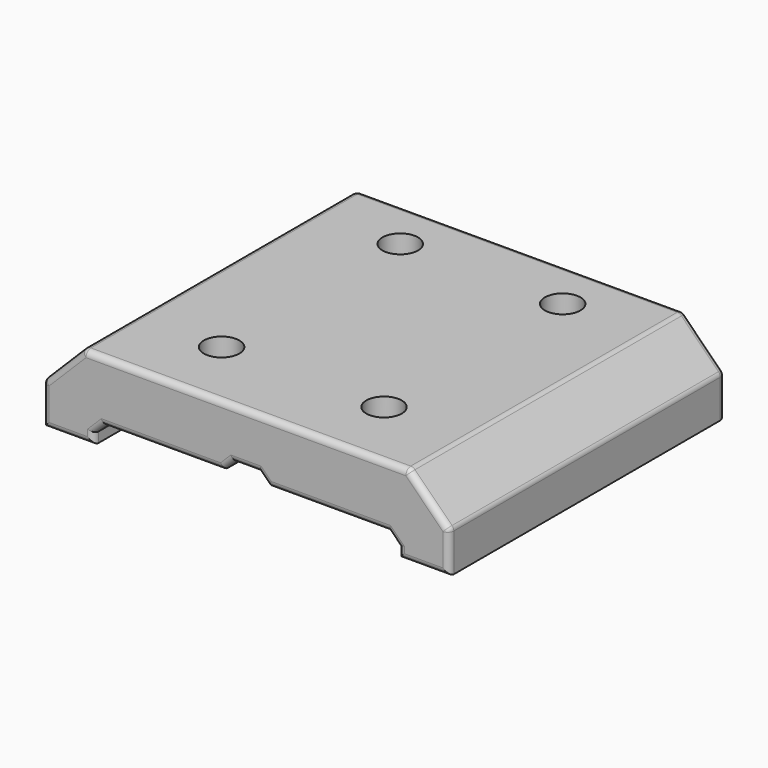
from build123d import *

# Parameters (mm, degrees)
F1_DEPTH = 34
F2_R     = 1.75
F3_DEPTH = 8.001
F4_SIZE  = 4
F5_SIZE  = 1
F8_R     = 0.6


with BuildPart() as f1:
    # F0 (on Front) → F1 (new body)
    with BuildSketch(Plane.XZ):
        Polygon((0, -5), (0, 0), (-20, 0), (-20, -8), (-15, -8), (-15, -6), (-2.2426406871, -6), (-1.2426406871, -5), align=None)
    extrude(amount=F1_DEPTH)

    # F2 (on face) → F3 (cut, through all)
    with BuildSketch(Plane.XY):
        with Locations((-8, -5)):
            Circle(F2_R)
        with Locations((-8, -27)):
            Circle(F2_R)
    extrude(amount=-F3_DEPTH, mode=Mode.SUBTRACT)

    # F4
    f4_edges = [f1.edges().sort_by_distance(p)[0] for p in [
        (-20, -17, 0),
    ]]
    chamfer(f4_edges, length=F4_SIZE)

    # F5
    f5_edges = [f1.edges().sort_by_distance(p)[0] for p in [
        (-15, -17, -6),
    ]]
    chamfer(f5_edges, length=F5_SIZE)

    # F6: F1 across face


with BuildPart() as f1_1:
    add(f1.part)
    add(f1.part.mirror(Plane(origin=(0, -17, -2.5), x_dir=(0, 1, 0), z_dir=(1, 0, 0))))

    # F8
    f8_edges = [f1_1.edges().sort_by_distance(p)[0] for p in [
        (20, -17, -4),
        (16, -17, 0),
        (-18, 0, -2),
        (-16, -17, 0),
        (-20, -17, -4),
        (-18, -34, -2),
        (-15, 0, -7.5),
        (-14.5, 0, -6.5),
        (-8.12132, 0, -6),
        (-1.742641, 0, -5.5),
        (0, 0, -5),
        (1.742641, 0, -5.5),
        (8.12132, 0, -6),
        (14.5, 0, -6.5),
        (15, 0, -7.5),
        (17.5, 0, -8),
        (20, 0, -6),
        (18, 0, -2),
        (0, 0, 0),
        (-20, 0, -6),
        (-17.5, 0, -8),
        (-17.5, -34, -8),
        (-15, -34, -7.5),
        (-14.5, -34, -6.5),
        (-8.12132, -34, -6),
        (-1.742641, -34, -5.5),
        (0, -34, -5),
        (1.742641, -34, -5.5),
        (8.12132, -34, -6),
        (14.5, -34, -6.5),
        (15, -34, -7.5),
        (17.5, -34, -8),
        (20, -34, -6),
        (18, -34, -2),
        (0, -34, 0),
        (-20, -34, -6),
    ]]
    fillet(f8_edges, radius=F8_R)


solid = f1_1.part
